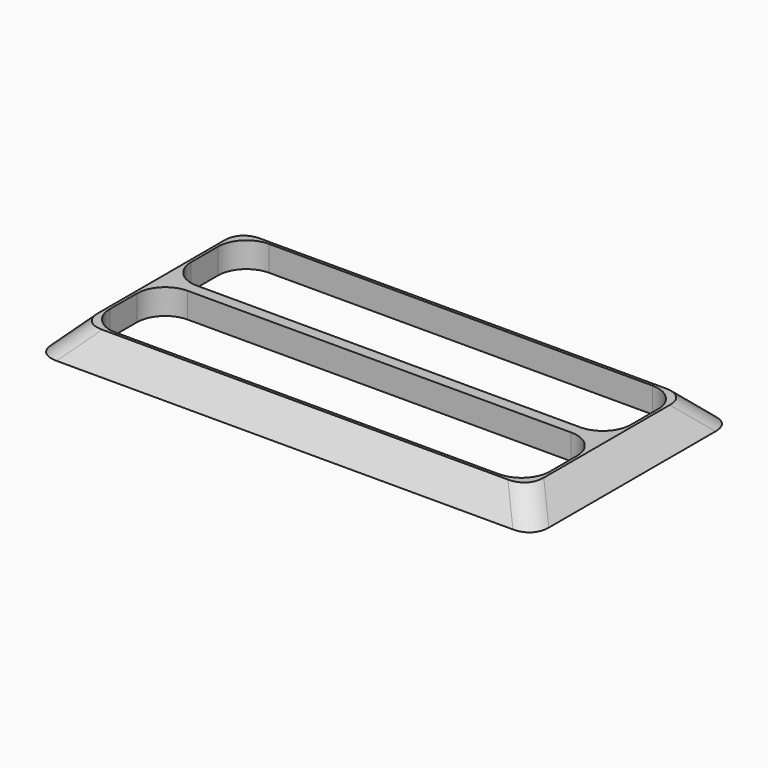
from build123d import *

# Parameters (mm, degrees)
F0_W        = 18
F0_H        = 9.2
F0_W_2      = 15.6
F0_H_2      = 3.2
F1_DEPTH    = 0.9
F2_T1_DEPTH = 23.6577025735
F2_T3_DEPTH = 14.8577025735
F3_R        = 1


# Not quite as in the source:
# - a fillet or chamfer that OpenCascade refuses, or shapes differently, is made with other operations: its cross-section is extruded or revolved along the edge and cut away or added


with BuildPart() as f1:
    # F0 (on Top) → F1 (new body)
    with BuildSketch(Plane.XY):
        Rectangle(F0_W, F0_H)
        with Locations((0, -1.8)):
            Rectangle(F0_W_2, F0_H_2, mode=Mode.SUBTRACT)
        with Locations((0, 1.8)):
            Rectangle(F0_W_2, F0_H_2, mode=Mode.SUBTRACT)
    extrude(amount=F1_DEPTH)

    # F2: chamfer of 1.1 on 4 edges, made by hand

    # F2_s2 → F2_t1 (cut)
    with BuildSketch(Plane.YZ.offset(-11.8288512868)):
        Polygon((-4.6, -0.2), (-3.5, 0.9), (-4.6, 0.9), align=None)
        Polygon((4.6, -0.2), (3.5, 0.9), (4.6, 0.9), align=None)
    extrude(amount=F2_T1_DEPTH, mode=Mode.SUBTRACT)

    # F2_s4 → F2_t3 (cut)
    with BuildSketch(Plane.XZ.offset(-7.4288512868)):
        Polygon((-9, -0.2), (-7.9, 0.9), (-9, 0.9), align=None)
        Polygon((9, -0.2), (7.9, 0.9), (9, 0.9), align=None)
    extrude(amount=F2_T3_DEPTH, mode=Mode.SUBTRACT)

    # F3
    f3_edges = [f1.edges().sort_by_distance(p)[0] for p in [
        (-7.8, 3.4, 0.45),
        (-7.8, -0.2, 0.45),
        (7.8, 0.2, 0.45),
        (7.8, -3.4, 0.45),
        (7.8, 3.4, 0.45),
        (7.8, -0.2, 0.45),
        (-7.8, 0.2, 0.45),
        (-7.8, -3.4, 0.45),
        (-8.35, -3.95, 0.45),
        (8.35, -3.95, 0.45),
        (8.35, 3.95, 0.45),
        (-8.35, 3.95, 0.45),
    ]]
    fillet(f3_edges, radius=F3_R)


solid = f1.part
